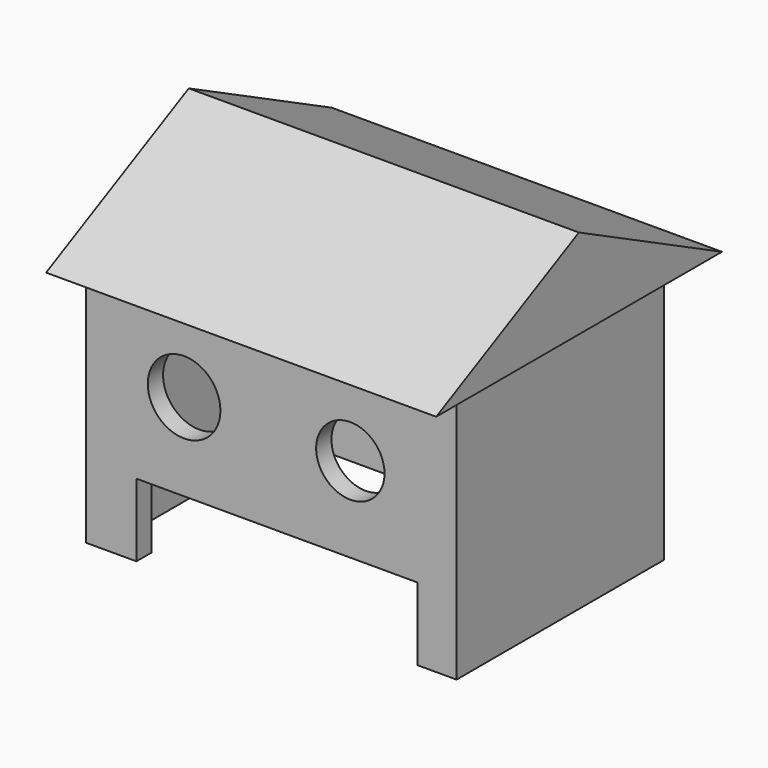
from build123d import *

# Parameters (mm, degrees)
F0_W          = 1724.6506214142
F0_H          = 612.7116954488
F0_W_2        = 1545.5847382545
F0_W_3        = 4094.7958827019
F0_W_4        = 7587.415933609
F0_H_2        = 515.1302540141
F0_W_5        = 442.0137703419
F0_H_3        = 2709.7913920879
F0_W_6        = 425.414532423
F0_H_4        = 1063.8439655304
F1_DEPTH      = 6940
F2_W          = 7587.415933609
F2_H          = 1964.671254158
F3_DEPTH      = 515.1302540141
F5_DEPTH      = 25
F5_DEPTH_BACK = 10500
F6_R          = 979.4636667312
F7_DEPTH      = 515.1302540141
F6_R_2        = 921.9518456682
F8_DEPTH      = 515.1312540141


# Not quite as in the source:
# - a feature names something its author has since deleted; it is built from what else it names


with BuildPart() as f1:
    # F0 (on Top) → F1 (new body)
    with BuildSketch(Plane.XY):
        Polygon((-3636.5358829498, 4472.7762019796), (-5000.3419220448, 4472.7762019796), (-5000.3419220448, 2272.7479934692), (-4558.3281517029, 2272.7479934692), (-4558.3281517029, 3860.0645065308), (-3636.5358829498, 3860.0645065308), align=None)
        with Locations((-2774.2105722427, 4166.4203542552)):
            Rectangle(F0_W, F0_H)
        with Locations((-1139.0928924084, 4166.4203542552)):
            Rectangle(F0_W_2, F0_H)
        Polygon((4999.6580779552, 4472.7762019796), (3728.4953594208, 4472.7762019796), (3728.4953594208, 3860.0645065308), (4574.2435455322, 3860.0645065308), (4574.2435455322, 2734.4160079956), (4999.6580779552, 2734.4160079956), align=None)
        Polygon((-4558.3281517029, -437.0433986187), (-5000.3419220448, -437.0433986187), (-5000.3419220448, -2527.2237980204), (-3638.1227970123, -2527.2237980204), (-3638.1227970123, -2012.0935440063), (-4558.3281517029, -2012.0935440063), align=None)
        Polygon((3949.2931365967, -2012.0935440063), (3949.2931365967, -2527.2237980204), (4999.6580779552, -2527.2237980204), (4999.6580779552, 1670.5720424652), (4574.2435455322, 1670.5720424652), (4574.2435455322, -2012.0935440063), align=None)
        with Locations((1681.0974180698, 4166.4203542552)):
            Rectangle(F0_W_3, F0_H)
        with Locations((155.5851697922, -2269.6586710134)):
            Rectangle(F0_W_4, F0_H_2)
        with Locations((-4779.3350368738, 917.8522974253)):
            Rectangle(F0_W_5, F0_H_3)
        with Locations((4786.9508117437, 2202.4940252304)):
            Rectangle(F0_W_6, F0_H_4)
    extrude(amount=F1_DEPTH)

    # F2 (on face) → F3 (cut, through all)
    with BuildSketch(Plane.XZ.offset(2527.2237980204)):
        with Locations((155.5851697922, 982.335627079)):
            Rectangle(F2_W, F2_H)
    extrude(amount=-F3_DEPTH, mode=Mode.SUBTRACT)

    # F4 (on face) → F5 (join, two sides)
    with BuildSketch(Plane(origin=(-5000.3419220448, 0, 0), x_dir=(0, -1, 0), z_dir=(-1, 0, 0))) as f5_sk:
        Polygon((-972.7762019796, 9359.9529266357), (-5797.1849441528, 6940), (-4472.7762019796, 6940), (2527.2237980204, 6940), (3838.9999866486, 6940), align=None)
    extrude(amount=F5_DEPTH)
    extrude(f5_sk.sketch, amount=-F5_DEPTH_BACK)

    # F6 (on face) → F7 (cut, through all)
    with BuildSketch(Plane.XZ.offset(2527.2237980204)):
        with Locations((-2351.0043621063, 4316.5826797485)):
            Circle(F6_R)
    extrude(amount=-F7_DEPTH, mode=Mode.SUBTRACT)

    # F6 (on face) → F8 (cut, through all)
    with BuildSketch(Plane.XZ.offset(2527.2237980204)):
        with Locations((-2351.0043621063, 4316.5826797485)):
            Circle(F6_R)
        with Locations((2133.8798999786, 4263.6985778809)):
            Circle(F6_R_2)
    extrude(amount=-F8_DEPTH, mode=Mode.SUBTRACT)


solid = f1.part
